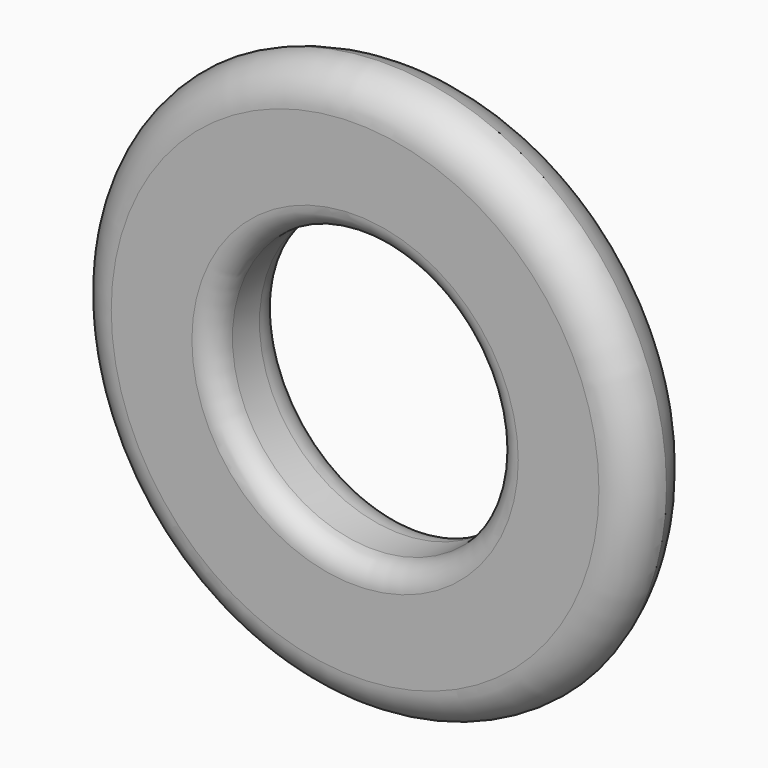
from build123d import *

# Parameters (mm, degrees)
F0_R     = 9.525
F0_R_2   = 4.7625
F1_DEPTH = 3.175
F2_R     = 1.27
F4_R     = 1.27
F5_R     = 0.762


# Not quite as in the source:
# - a fillet or chamfer that OpenCascade refuses, or shapes differently, is made with other operations: its cross-section is extruded or revolved along the edge and cut away or added


with BuildPart() as f1:
    # F0 (on Front) → F1 (new body)
    with BuildSketch(Plane.XZ):
        Circle(F0_R)
        Circle(F0_R_2, mode=Mode.SUBTRACT)
    extrude(amount=F1_DEPTH)

    # F2
    f2_edges = [f1.edges().sort_by_distance(p)[0] for p in [
        (-9.525, -3.175, 0),
    ]]
    fillet(f2_edges, radius=F2_R)

    # F3: fillet of radius 2.54 on 1 edges, made by hand

    # F3_s1 → F3_t2 (revolve, cut)
    with BuildSketch(Plane.XY):
        with BuildLine():
            ThreePointArc((9.525, -1.905), (8.6210815618, -0.5319536858), (7.0656555752, 0))
            Line((7.0656555752, 0), (7.0656555752, 0.0508))
            Line((7.0656555752, 0.0508), (9.525, 0.0508))
            Line((9.525, 0.0508), (9.5758, 0))
            ThreePointArc((9.5758, 0), (9.5758, -0.9525), (9.5741868885, -1.8923))
            Line((9.5741868885, -1.8923), (9.525, -1.905))
        make_face()
    revolve(axis=Axis((0, 0, 0), (0, -1, 0)), mode=Mode.SUBTRACT)

    # F4
    f4_edges = [f1.edges().sort_by_distance(p)[0] for p in [
        (-4.7625, 0, 0),
    ]]
    fillet(f4_edges, radius=F4_R)

    # F5
    f5_edges = [f1.edges().sort_by_distance(p)[0] for p in [
        (-4.7625, -3.175, 0),
    ]]
    fillet(f5_edges, radius=F5_R)


solid = f1.part
